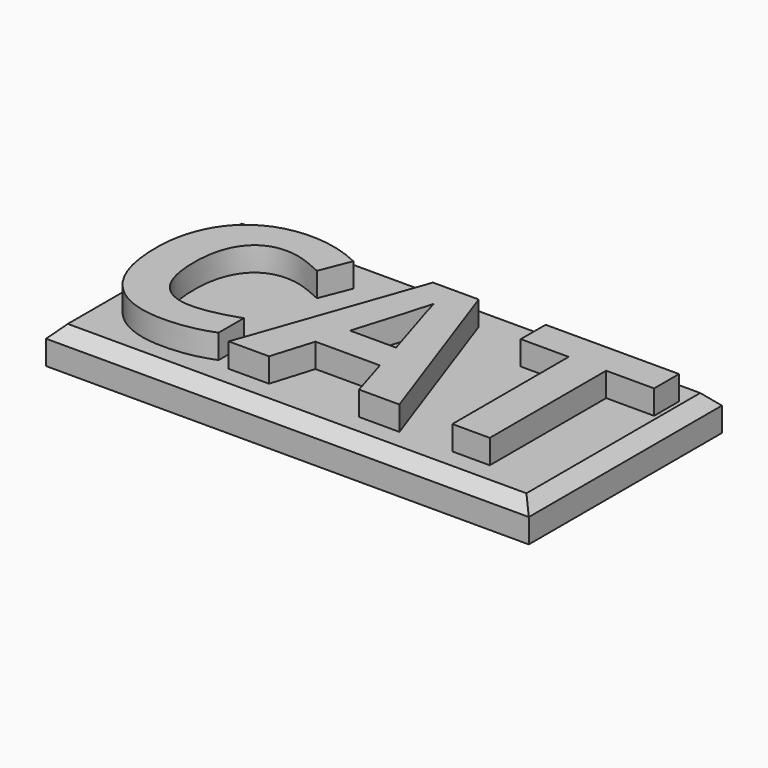
from build123d import *

# Parameters (mm, degrees)
F0_W         = 40
F0_H         = 20
F1_DEPTH     = 3
F2_TEXT_SIZE = 20.5013213742
F3_DEPTH     = 2
F4_SIZE      = 1


# Not quite as in the source:
# - Text() gives the source's letters only with a copy of the font that has no kerning and outlines rounded to 1/6400 em; it was checked with that copy


with BuildPart() as f1:
    # F0 (on Top) → F1 (new body)
    with BuildSketch(Plane.XY):
        Rectangle(F0_W, F0_H)
    extrude(amount=F1_DEPTH)

    # F2 (on face) → F3 (join)
    with BuildSketch(Plane.XY.offset(3)):
        with Locations((-20, -7.41689555)):
            Text('CAT', F2_TEXT_SIZE, font='Open Sans', font_style=FontStyle.BOLD, text_align=(TextAlign.LEFT, TextAlign.BOTTOM))
    extrude(amount=F3_DEPTH)

    # F4
    f4_edges = [f1.edges().sort_by_distance(p)[0] for p in [
        (-20, 0, 3),
        (0, -10, 3),
        (20, 0, 3),
        (0, 10, 3),
    ]]
    chamfer(f4_edges, length=F4_SIZE)


solid = f1.part
